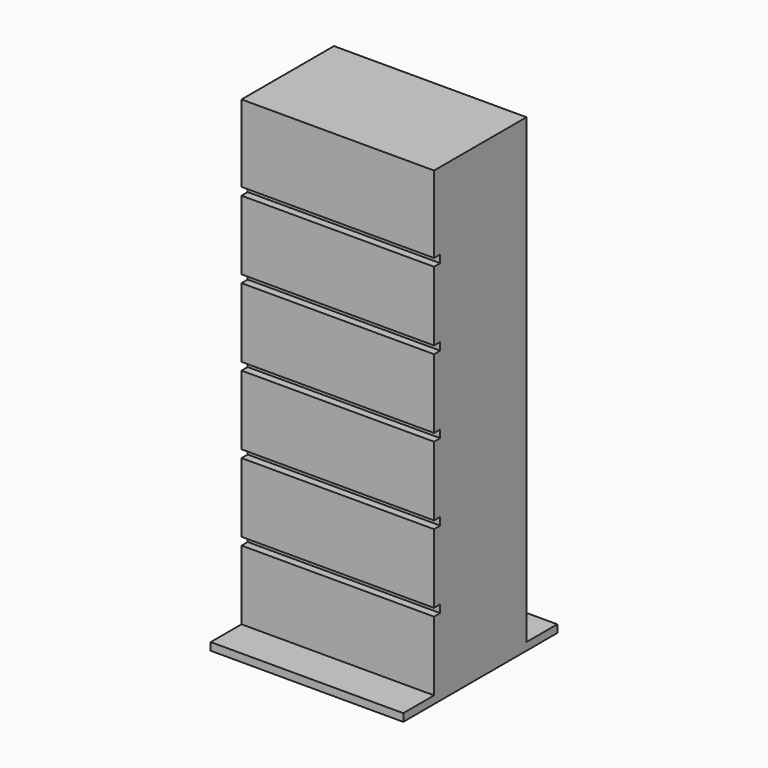
from build123d import *

# Parameters (mm, degrees)
F0_W         = 25
F0_H         = 25
F1_DEPTH     = 1
F2_W         = 25
F2_H         = 15
F3_DEPTH     = 60
F4_W         = 1
F4_H         = 1
F5_DEPTH     = 25.001
F6_TEXT_SIZE = 12.5
F7_DEPTH     = 1


# Not quite as in the source:
# - Text() gives the source's letters only with a copy of the font that has no kerning and outlines rounded to 1/6400 em; it was checked with that copy


with BuildPart() as f1:
    # F0 (on Top) → F1 (new body)
    with BuildSketch(Plane.XY):
        Rectangle(F0_W, F0_H)
    extrude(amount=F1_DEPTH)

    # F2 (on face) → F3 (join)
    with BuildSketch(Plane.XY.offset(1)):
        Rectangle(F2_W, F2_H)
    extrude(amount=F3_DEPTH)

    # F4 (on face) → F5 (cut, through all)
    with BuildSketch(Plane(origin=(-12.5, 0, 0), x_dir=(0, -1, 0), z_dir=(-1, 0, 0))):
        with Locations((7, 50.5)):
            Rectangle(F4_W, F4_H)
        with Locations((7, 40.5)):
            Rectangle(F4_W, F4_H)
        with Locations((7, 30.5)):
            Rectangle(F4_W, F4_H)
        with Locations((7, 20.5)):
            Rectangle(F4_W, F4_H)
        with Locations((7, 10.5)):
            Rectangle(F4_W, F4_H)
    extrude(amount=-F5_DEPTH, mode=Mode.SUBTRACT)

    # F6 (on face) → F7 (cut)
    with BuildSketch(Plane(origin=(0, 7.5, 0), x_dir=(-1, 0, 0), z_dir=(0, 1, 0))):
        with Locations((-2.5869140625, 1)):
            Text('1', F6_TEXT_SIZE, font='Open Sans', text_align=(TextAlign.LEFT, TextAlign.BOTTOM))
        with Locations((-3.6435546875, 11)):
            Text('2', F6_TEXT_SIZE, font='Open Sans', text_align=(TextAlign.LEFT, TextAlign.BOTTOM))
        with Locations((-3.853515625, 31)):
            Text('4', F6_TEXT_SIZE, font='Open Sans', text_align=(TextAlign.LEFT, TextAlign.BOTTOM))
        with Locations((-3.619140625, 41)):
            Text('5', F6_TEXT_SIZE, font='Open Sans', text_align=(TextAlign.LEFT, TextAlign.BOTTOM))
        with Locations((-3.673828125, 51)):
            Text('6', F6_TEXT_SIZE, font='Open Sans', text_align=(TextAlign.LEFT, TextAlign.BOTTOM))
        with Locations((-3.6123046875, 21)):
            Text('3', F6_TEXT_SIZE, font='Open Sans', text_align=(TextAlign.LEFT, TextAlign.BOTTOM))
    extrude(amount=-F7_DEPTH, mode=Mode.SUBTRACT)


solid = f1.part
